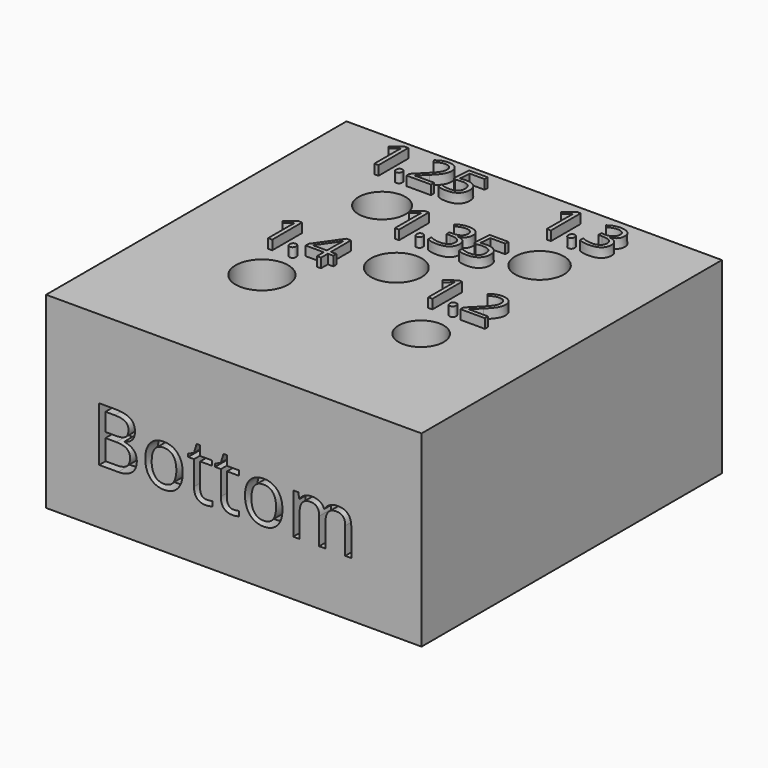
from build123d import *

# Parameters (mm, degrees)
F0_W         = 10
F0_H         = 10
F1_DEPTH     = 5
F2_R         = 0.6
F2_R_2       = 0.675
F2_R_3       = 0.7
F2_R_4       = 0.625
F2_R_5       = 0.65
F5_DEPTH     = 25
F3_TEXT_SIZE = 2.6078461411
F6_DEPTH     = 0.4
F4_TEXT_SIZE = 2.0277587787
F7_DEPTH     = 0.4
F2_TEXT_SIZE = 1.3888888889
F8_DEPTH     = 0.25


# Not quite as in the source:
# - Text() gives the source's letters only with a copy of the font that has no kerning and outlines rounded to 1/6400 em; it was checked with that copy


with BuildPart() as f1:
    # F0 (on Top) → F1 (new body)
    with BuildSketch(Plane.XY):
        with Locations((-0.6542224437, -2.4417747585)):
            Rectangle(F0_W, F0_H)
    extrude(amount=F1_DEPTH)

    # F2 (on face) → F5 (cut)
    with BuildSketch(Plane.XY.offset(5)):
        with Locations((1.5353794525, -3.9417747585)):
            Circle(F2_R)
        with Locations((-0.7263370873, -1.9417747585)):
            Circle(F2_R_2)
        with Locations((-2.7053392609, -3.9417747585)):
            Circle(F2_R_3)
        with Locations((-2.7053392609, 0.0582252415)):
            Circle(F2_R_4)
        with Locations((1.5353794525, 0)):
            Circle(F2_R_5)
    extrude(amount=-F5_DEPTH, mode=Mode.SUBTRACT)

    # F3 (on face) → F6 (join)
    with BuildSketch(Plane(origin=(0, 2.5582252415, 0), x_dir=(-1, 0, 0), z_dir=(0, 1, 0))):
        with Locations((-1.7075833166, 1.4582271688)):
            Text('Top', F3_TEXT_SIZE, font='Open Sans', text_align=(TextAlign.LEFT, TextAlign.BOTTOM))
    extrude(amount=F6_DEPTH)

    # F4 (on face) → F7 (cut)
    with BuildSketch(Plane.XZ.offset(7.4417747585)):
        with Locations((-4.4400414045, 1.4679984888)):
            Text('Bottom', F4_TEXT_SIZE, font='Open Sans', text_align=(TextAlign.LEFT, TextAlign.BOTTOM))
    extrude(amount=-F7_DEPTH, mode=Mode.SUBTRACT)

    # F2 (on face) → F8 (join)
    with BuildSketch(Plane.XY.offset(5)):
        with Locations((-4.0863071429, 1.0582252415)):
            Text('1.25', F2_TEXT_SIZE, font='Open Sans', text_align=(TextAlign.LEFT, TextAlign.BOTTOM))
        with Locations((0.5521980289, 1)):
            Text('1.3', F2_TEXT_SIZE, font='Open Sans', text_align=(TextAlign.LEFT, TextAlign.BOTTOM))
        with Locations((-1.9386824242, -0.9417747585)):
            Text('1.35', F2_TEXT_SIZE, font='Open Sans', text_align=(TextAlign.LEFT, TextAlign.BOTTOM))
        with Locations((0.5487258067, -2.9417747585)):
            Text('1.2', F2_TEXT_SIZE, font='Open Sans', text_align=(TextAlign.LEFT, TextAlign.BOTTOM))
        with Locations((-3.7153218998, -2.9417747585)):
            Text('1.4', F2_TEXT_SIZE, font='Open Sans', text_align=(TextAlign.LEFT, TextAlign.BOTTOM))
    extrude(amount=F8_DEPTH)


solid = f1.part
